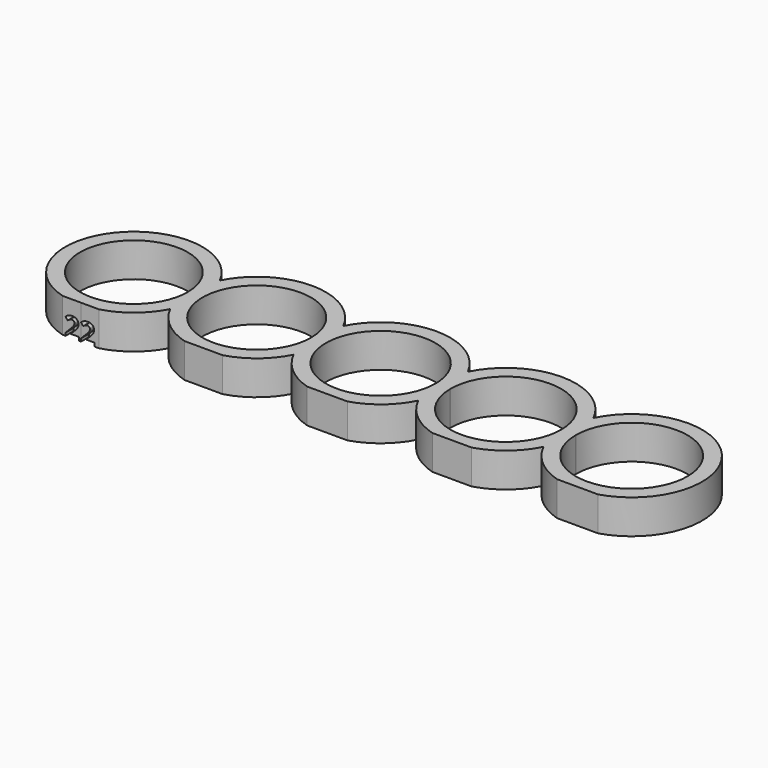
from build123d import *

# Parameters (mm, degrees)
F0_R         = 11
F0_R_2       = 11.1
F1_DEPTH     = 7
F3_DEPTH     = 25
F4_TEXT_SIZE = 5.5555555556
F5_DEPTH     = 2


# Not quite as in the source:
# - Text() gives the source's letters only with a copy of the font that has no kerning and outlines rounded to 1/6400 em; it was checked with that copy


with BuildPart() as f1:
    # F0 (on Top) → F1 (new body)
    with BuildSketch(Plane.XY):
        with BuildLine():
            ThreePointArc((-12.7059288538, 6.3402974665), (-25.3132623168, 14.0999937628), (-37.9059760956, 6.3165945474))
            ThreePointArc((-37.9059760956, 6.3165945474), (-64.4, 0), (-37.9059760956, -6.3165945474))
            ThreePointArc((-37.9059760956, -6.3165945474), (-25.3132623168, -14.0999937628), (-12.7059288538, -6.3402974665))
            ThreePointArc((-12.7059288538, -6.3402974665), (0.0106309316, -14.1999960205), (12.7154080262, -6.3212655955))
            ThreePointArc((12.7154080262, -6.3212655955), (25.5100896394, -14.2141725597), (38.2933355698, -6.3027579318))
            ThreePointArc((38.2933355698, -6.3027579318), (65.5991009343, 0.0842659381), (38.2938318917, 6.4734113087))
            ThreePointArc((38.2938318917, 6.4734113087), (25.4625163139, 14.3857752427), (12.6725698607, 6.4067131297))
            ThreePointArc((12.6725698607, 6.4067131297), (-0.0371613467, 14.1999513744), (-12.7059288538, 6.3402974665))
        make_face()
        with Locations((-50.4, 0)):
            Circle(F0_R, mode=Mode.SUBTRACT)
        with Locations((-25.3, 0)):
            Circle(F0_R_2, mode=Mode.SUBTRACT)
        with BuildLine():
            ThreePointArc((11.1997462617, 0.0753901352), (11.1999365653, 0.0376952811), (11.2, 0))
            ThreePointArc((11.2, 0), (-11.1999365653, -0.0376952811), (11.1997462617, 0.0753901352))
        make_face(mode=Mode.SUBTRACT)
        with BuildLine():
            ThreePointArc((36.7993865126, 0.1755130587), (36.7996534694, 0.1306687309), (36.7997424555, 0.0858236968))
            ThreePointArc((36.7997424555, 0.0858236968), (36.7996517188, 0.0405396898), (36.7993795101, -0.00474359))
            ThreePointArc((36.7993795101, -0.00474359), (25.4923396063, -11.2141738783), (14.1999964353, 0.0100617075))
            ThreePointArc((14.1999964353, 0.0100617075), (14.1999195738, 0.0477922314), (14.1997424595, 0.085522418))
            ThreePointArc((14.1997424595, 0.085522418), (25.4547467832, 11.3857341119), (36.7993865126, 0.1755130587))
        make_face(mode=Mode.SUBTRACT)
        with BuildLine():
            ThreePointArc((39.7994613977, 0.1754795622), (51.2444284137, 11.4847352282), (62.5991009451, 0.0848253417))
            ThreePointArc((62.5991009451, 0.0848253417), (51.243985556, -11.315086297), (39.7994543887, -0.0049431841))
            ThreePointArc((39.7994543887, -0.0049431841), (39.7991009538, 0.0852682029), (39.7994613977, 0.1754795622))
        make_face(mode=Mode.SUBTRACT)
    extrude(amount=F1_DEPTH)

    # F2 (on face) → F3 (cut)
    with BuildSketch(Plane.XY.offset(7)):
        Polygon((63.8250187039, -13.7141725597), (-50.3988280685, -13.5000013734), (-55.8023605749, -13.4898696803), (-55.8023605749, -17.6281966269), (63.8250187039, -17.8524995063), align=None)
    extrude(amount=-F3_DEPTH, mode=Mode.SUBTRACT)

    # F4 (on face) → F5 (cut)
    with BuildSketch(Plane(origin=(-0.0254897729, -13.5944520326, 0), x_dir=(0.9999982422, -0.0018750096, 0), z_dir=(-0.0018750096, -0.9999982422, 0))):
        with Locations((-53.7634752691, 0)):
            Text('22', F4_TEXT_SIZE, font='Open Sans', font_style=FontStyle.BOLD, text_align=(TextAlign.LEFT, TextAlign.BOTTOM))
    extrude(amount=-F5_DEPTH, mode=Mode.SUBTRACT)


solid = f1.part
